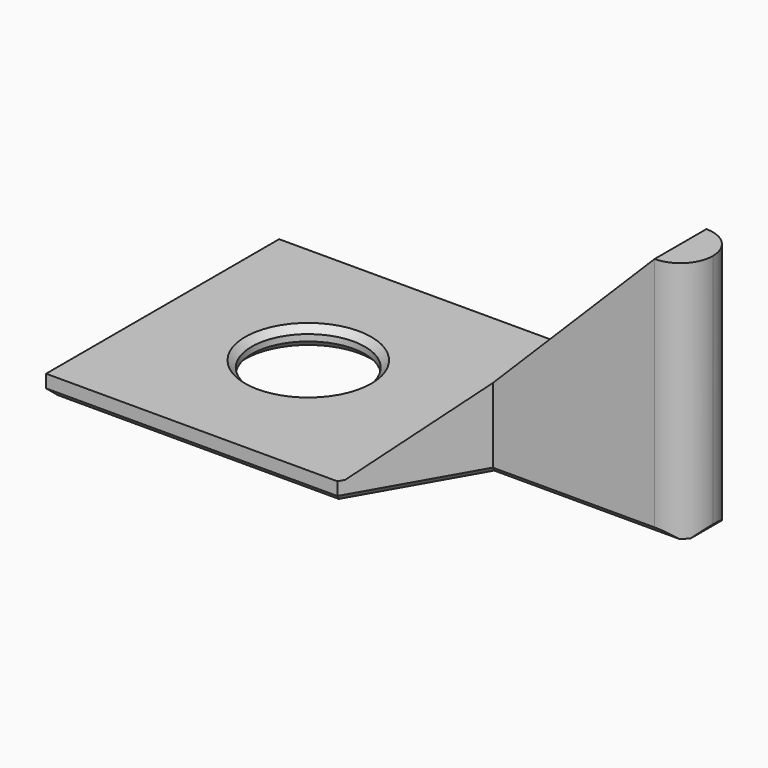
from build123d import *

# Parameters (mm, degrees)
F0_W        = 18
F0_H        = 18
F0_R        = 3.5
F1_DEPTH    = 1.2
F3_DEPTH    = 15
F4_T4_DEPTH = 90.007123663
F5_SIZE     = 0.4
F6_T1_DEPTH = 24.6


# Not quite as in the source:
# - a fillet or chamfer that OpenCascade refuses, or shapes differently, is made with other operations: its cross-section is extruded or revolved along the edge and cut away or added


with BuildPart() as f1:
    # F0 (on Top) → F1 (new body)
    with BuildSketch(Plane.XY):
        Rectangle(F0_W, F0_H)
        Circle(F0_R, mode=Mode.SUBTRACT)
    extrude(amount=F1_DEPTH)

    # F2 (on face) → F3 (join)
    with BuildSketch(Plane(origin=(0, 0, 0), x_dir=(1, 0, 0), z_dir=(0, 0, -1))):
        Polygon((9, 0), (9, -9), (13, -2), (25, -2), (25, 0), align=None)
        Polygon((9, 9), (9, 0), (25, 0), (25, 2), (13, 2), align=None)
    extrude(amount=-F3_DEPTH)

    # F4: chamfer of 14 on 1 edges, made by hand


with BuildPart() as f4_tool2:
    # F4_s3 → F4_t4 (new body)
    with BuildSketch(Plane.XZ.offset(45.0035618315)):
        Polygon((9, 1), (23, 15), (9, 15), align=None)
    extrude(amount=-F4_T4_DEPTH)

    split(bisect_by=Plane.XY.offset(1.2), keep=Keep.TOP)


with BuildPart() as f1_1:
    add(f1.part)

    # F4_t1: cut F4_tool2
    add(f4_tool2.part, mode=Mode.SUBTRACT)

    # F5
    f5_edges = [f1_1.edges().sort_by_distance(p)[0] for p in [
        (0, -9, 0),
        (11, -5.5, 0),
        (19, -2, 0),
        (25, 0, 0),
        (19, 2, 0),
        (11, 5.5, 0),
        (0, 9, 0),
        (-9, 0, 0),
        (-3.5, 0, 0),
        (-3.5, 0, 1.2),
    ]]
    chamfer(f5_edges, length=F5_SIZE)

    # F6: fillet of radius 2 on 2 edges, made by hand

    # F6_s2 → F6_t1 (cut)
    with BuildSketch(Plane.XY.offset(-4.6)):
        with BuildLine():
            ThreePointArc((23, -2), (24.4142135624, -1.4142135624), (25, 0))
            Line((25, 0), (25, -2))
            Line((25, -2), (23, -2))
        make_face()
        with BuildLine():
            ThreePointArc((23, 2), (24.4142135624, 1.4142135624), (25, 0))
            Line((25, 0), (25, 2))
            Line((25, 2), (23, 2))
        make_face()
    extrude(amount=F6_T1_DEPTH, mode=Mode.SUBTRACT)


solid = f1_1.part
